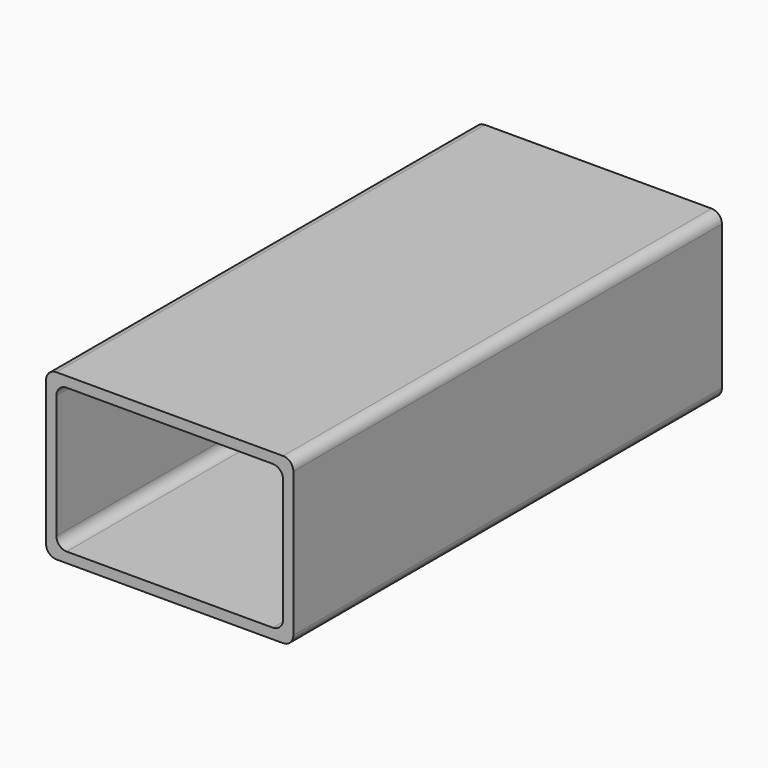
from build123d import *

# Parameters (mm, degrees)
F0_W     = 76.2
F0_H     = 50.8
F0_W_2   = 69.85
F0_H_2   = 44.45
F2_DEPTH = 165.1
F3_R     = 3.175


# Not quite as in the source:
# - a variable given as a bare number and used for a length is read in inches; the dataset says mm whatever the document's units were


with BuildPart() as f2:
    # F0 (on Front) → F2 (new body)
    with BuildSketch(Plane.XZ):
        Rectangle(F0_W, F0_H)
        Rectangle(F0_W_2, F0_H_2, mode=Mode.SUBTRACT)
    extrude(amount=F2_DEPTH)

    # F3
    f3_edges = [f2.edges().sort_by_distance(p)[0] for p in [
        (-34.925, -82.55, 22.225),
        (34.925, -82.55, 22.225),
        (34.925, -82.55, -22.225),
        (-34.925, -82.55, -22.225),
        (38.1, -82.55, 25.4),
        (38.1, -82.55, -25.4),
        (-38.1, -82.55, -25.4),
        (-38.1, -82.55, 25.4),
    ]]
    fillet(f3_edges, radius=F3_R)


solid = f2.part
